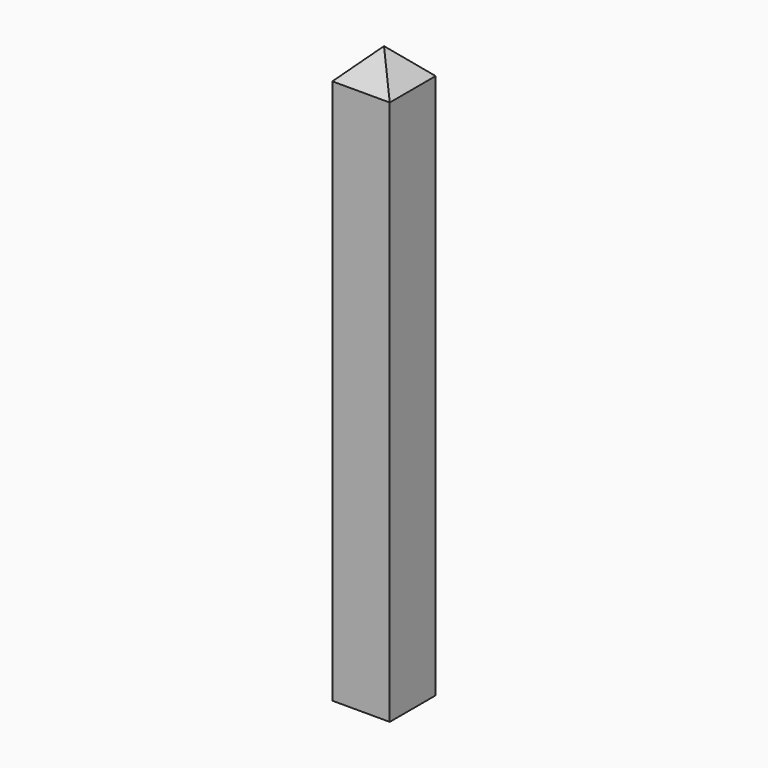
from build123d import *

# Parameters (mm, degrees)
F0_W     = 12.7
F0_H     = 12.7
F1_DEPTH = 127
F2_SIZE  = 6.34999


# Not quite as in the source:
# - a fillet or chamfer is up to 0.001 mm smaller than in the source, because OpenCascade refuses the exact size


with BuildPart() as f1:
    # F0 (on Top) → F1 (new body)
    with BuildSketch(Plane.XY):
        with Locations((-30.6644180454, -5.2849810437)):
            Rectangle(F0_W, F0_H)
    extrude(amount=F1_DEPTH)

    # F2 (size 6.35 in the source; OpenCascade refuses exactly that, so slightly less here)
    f2_edges = [f1.edges().sort_by_distance(p)[0] for p in [
        (-37.014418, -5.284981, 127),
        (-24.314418, -5.284981, 127),
        (-30.664418, -11.634981, 127),
        (-30.664418, 1.065019, 127),
    ]]
    chamfer(f2_edges, length=F2_SIZE)


solid = f1.part
